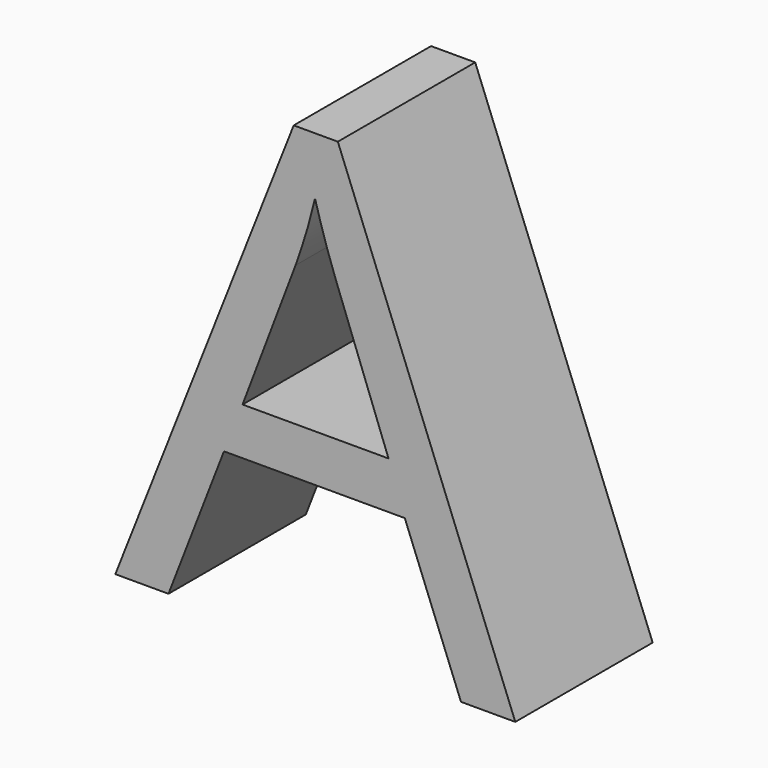
from build123d import *

# Parameters (mm, degrees)
F0_TEXT_SIZE = 92.0227780524
F1_DEPTH     = 25


# Not quite as in the source:
# - Text() gives the source's letters only with a copy of the font that has no kerning and outlines rounded to 1/6400 em; it was checked with that copy


with BuildPart() as f1:
    # F0 (on Front) → F1 (new body)
    with BuildSketch(Plane.XZ):
        with Locations((-43.6067059636, -25.2306982875)):
            Text('A', F0_TEXT_SIZE, font='Open Sans', text_align=(TextAlign.LEFT, TextAlign.BOTTOM))
    extrude(amount=-F1_DEPTH)


solid = f1.part
